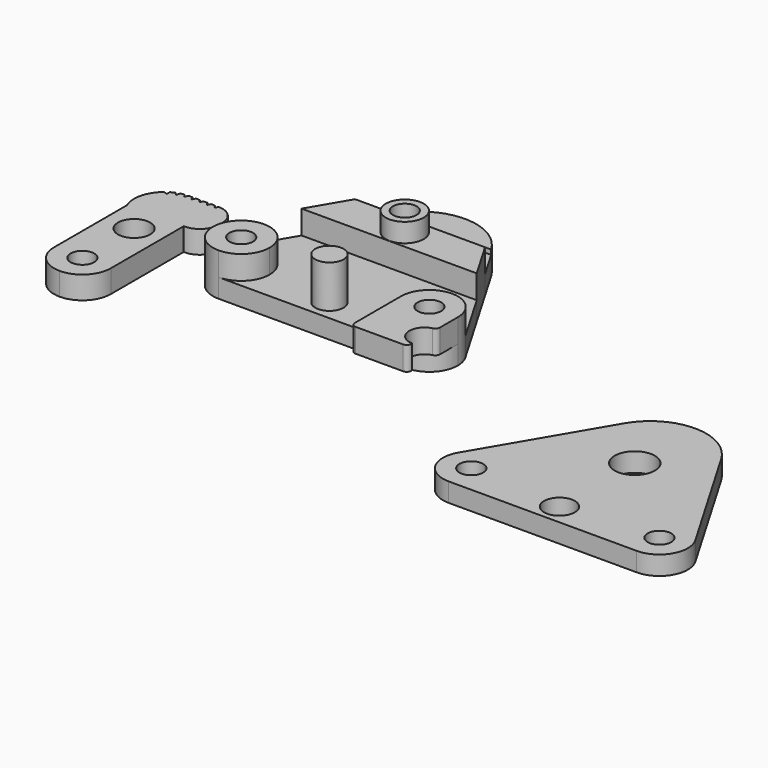
from build123d import *

# Parameters (mm, degrees)
F0_R            = 3.81
F2_DEPTH        = 5.08
F0_R_2          = 5.08
F0_R_3          = 3.175
F3_DEPTH        = 11.43
F4_DEPTH        = 16.51
F5_DEPTH        = 6.35
F6_START        = 5.08
F6_DEPTH        = 6.35
F1_R            = 3.175
F1_R_2          = 4.318
F7_DEPTH        = 6.096
F8_R            = 3.175
F8_R_2          = 4.1275
F8_R_3          = 5.3975
F9_DEPTH        = 5.08
F10_D           = 6.35
F10_CBORE_D     = 12.7
F10_CBORE_DEPTH = 3.81


# Not quite as in the source:
# - a feature names something its author has since deleted; it is built from what else it names


with BuildPart() as f2:
    # F0 (on Top) → F2 (new body)
    with BuildSketch(Plane.XY):
        with BuildLine():
            ThreePointArc((-17.6954780992, -30.626333441), (-19.9273244266, -36.0144871136), (-25.3154780992, -38.246333441))
            Line((-25.3154780992, -38.246333441), (17.5577984688, -38.246333441))
            Line((17.5577984688, -38.246333441), (17.5577984688, -30.626333441))
            ThreePointArc((17.5577984688, -30.626333441), (23.1855190024, -23.271387994), (31.7560196047, -26.7803736534))
            Line((31.7560196047, -26.7803736534), (23.4553135122, -12.5826484363))
            Line((23.4553135122, -12.5826484363), (-23.5570166859, -12.5826484363))
            Line((-23.5570166859, -12.5826484363), (-31.8864294526, -26.7679661294))
            ThreePointArc((-31.8864294526, -26.7679661294), (-23.3162594159, -23.2732711771), (-17.6954780992, -30.626333441))
        make_face()
        with Locations((0, -32.6841548085)):
            Circle(F0_R, mode=Mode.SUBTRACT)
        with BuildLine():
            Line((17.5577984688, -30.626333441), (17.5577984688, -38.246333441))
            Line((17.5577984688, -38.246333441), (25.1777984688, -38.246333441))
            ThreePointArc((25.1777984688, -38.246333441), (19.7896447962, -36.0144871136), (17.5577984688, -30.626333441))
        make_face()
    extrude(amount=F2_DEPTH)



with BuildPart() as f2b:
    # F0 (on Top) → F2, piece 2 (new body)
    with BuildSketch(Plane.XY):
        Polygon((-13.0052492681, 5.3874266745), (-17.4796027267, -2.2325733255), (17.4113143411, -2.2448484363), (12.9634277073, 5.3629227003), align=None)
    extrude(amount=F2_DEPTH)


with BuildPart() as f2_1:
    add(f2.part)

    add(f2b.part)  # F3 merges F2b
    # F0 (on Top) → F3 (join)
    with BuildSketch(Plane.XY):
        Polygon((-17.4796027267, -2.2325733255), (-23.5570166859, -12.5826484363), (23.4553135122, -12.5826484363), (17.4113143411, -2.2448484363), align=None)
        with Locations((0, -7.4137484363)):
            Circle(F0_R_2, mode=Mode.SUBTRACT)
        with BuildLine():
            ThreePointArc((-31.8864294526, -26.7679661294), (-31.9285393765, -34.4120725422), (-25.3154780992, -38.246333441))
            ThreePointArc((-25.3154780992, -38.246333441), (-19.9273244266, -36.0144871136), (-17.6954780992, -30.626333441))
            ThreePointArc((-17.6954780992, -30.626333441), (-23.3162594159, -23.2732711771), (-31.8864294526, -26.7679661294))
        make_face()
        with Locations((-25.3154780992, -30.626333441)):
            Circle(F0_R_3, mode=Mode.SUBTRACT)
        with BuildLine():
            ThreePointArc((17.5577984688, -30.626333441), (19.7896447962, -36.0144871136), (25.1777984688, -38.246333441))
            ThreePointArc((25.1777984688, -38.246333441), (30.5659521415, -36.0144871136), (32.7977984688, -30.626333441))
            ThreePointArc((32.7977984688, -30.626333441), (32.5327439158, -28.6340539746), (31.7560196047, -26.7803736534))
            ThreePointArc((31.7560196047, -26.7803736534), (23.1855190024, -23.271387994), (17.5577984688, -30.626333441))
        make_face()
        with Locations((25.1777984688, -30.626333441)):
            Circle(F0_R_3, mode=Mode.SUBTRACT)
        with BuildLine():
            Line((17.5577984688, -30.626333441), (17.5577984688, -38.246333441))
            Line((17.5577984688, -38.246333441), (25.1777984688, -38.246333441))
            ThreePointArc((25.1777984688, -38.246333441), (19.7896447962, -36.0144871136), (17.5577984688, -30.626333441))
        make_face()
        with Locations((25.1777984688, -30.626333441)):
            Circle(F0_R_3)
        with Locations((-25.3154780992, -30.626333441)):
            Circle(F0_R_3)
    extrude(amount=F3_DEPTH)

    # F0 (on Top) → F4 (join)
    with BuildSketch(Plane.XY):
        with Locations((0, -32.6841548085)):
            Circle(F0_R)
        with Locations((0, -7.4137484363)):
            Circle(F0_R_2)
        with Locations((0, -7.4137484363)):
            Circle(F0_R_3, mode=Mode.SUBTRACT)
        with Locations((0, -7.4137484363)):
            Circle(F0_R_3)
    extrude(amount=F4_DEPTH)

    # F0 (on Top) → F5 (join)
    with BuildSketch(Plane.XY):
        with BuildLine():
            ThreePointArc((12.9634277073, 5.3629227003), (-0.0138892827, 12.8163759997), (-13.0052492681, 5.3874266745))
            Line((-13.0052492681, 5.3874266745), (12.9634277073, 5.3629227003))
        make_face()
    extrude(amount=F5_DEPTH)

    # F0 (on Top) → F6 (join)
    with BuildSketch(Plane.XY.offset(F6_START)):
        with BuildLine():
            Line((25.1777984688, -38.246333441), (17.5577984688, -38.246333441))
            Line((17.5577984688, -38.246333441), (17.5577984688, -46.1423077567))
            ThreePointArc((17.5577984688, -46.1423077567), (17.9297728567, -47.0403333688), (18.8277984688, -47.4123077567))
            Line((18.8277984688, -47.4123077567), (31.5277984688, -47.4123077567))
            ThreePointArc((31.5277984688, -47.4123077567), (32.4258240809, -47.0403333688), (32.7977984688, -46.1423077567))
            Line((32.7977984688, -46.1423077567), (32.7977984688, -46.0876021411))
            ThreePointArc((32.7977984688, -46.0876021411), (32.7285996668, -45.9133479668), (32.5587077819, -45.8340400927))
            ThreePointArc((32.5587077819, -45.8340400927), (28.7412851246, -42.1364642502), (31.8296571838, -37.8113352487))
            ThreePointArc((31.8296571838, -37.8113352487), (32.5268631734, -37.3618027602), (32.7977984688, -36.5777302406))
            Line((32.7977984688, -36.5777302406), (32.7977984688, -30.626333441))
            ThreePointArc((32.7977984688, -30.626333441), (30.5659521415, -36.0144871136), (25.1777984688, -38.246333441))
        make_face()
    extrude(amount=F6_DEPTH)

    # F10 (through all)
    with Locations(Plane(origin=(0, 0, 0), x_dir=(1, 0, 0), z_dir=(0, 0, -1))):
        with Locations((-25.3154780992, 30.626333441), (25.1777984688, 30.626333441), (0, 7.4137484363)):
            CounterBoreHole(F10_D / 2, F10_CBORE_D / 2, F10_CBORE_DEPTH)


with BuildPart() as f7:
    # F1 (on face) → F7 (new body)
    with BuildSketch(Plane.XY):
        with BuildLine():
            ThreePointArc((-57.1931454593, -16.6974549338), (-59.9398799438, -21.0814893724), (-59.5037853794, -26.2364995391))
            Line((-59.5037853794, -26.2364995391), (-44.4651611469, -26.2364995391))
            Line((-44.4651611469, -26.2364995391), (-44.2637853794, -26.2364995391))
            Line((-44.2637853794, -26.2364995391), (-44.0075451514, -26.2364995391))
            ThreePointArc((-44.0075451514, -26.2364995391), (-40.415442703, -24.7486019875), (-38.9275451514, -21.1564995391))
            Line((-38.9275451514, -21.1564995391), (-38.9275451514, -19.9137048024))
            ThreePointArc((-38.9275451514, -19.9137048024), (-40.4075319267, -16.3295305904), (-43.9851454593, -14.8337541872))
            Line((-43.9851454593, -14.8337541872), (-44.4931882277, -15.7136113037))
            Line((-44.4931882277, -15.7136113037), (-45.0011454593, -14.8337048024))
            Line((-45.0011454593, -14.8337048024), (-46.0171454593, -14.8337048024))
            Line((-46.0171454593, -14.8337048024), (-46.5251454593, -15.7135866127))
            Line((-46.5251454593, -15.7135866127), (-47.0331454593, -14.8337048024))
            Line((-47.0331454593, -14.8337048024), (-48.0491454593, -14.8337048024))
            Line((-48.0491454593, -14.8337048024), (-48.5571454593, -15.7135866127))
            Line((-48.5571454593, -15.7135866127), (-49.0651454593, -14.8337048024))
            Line((-49.0651454593, -14.8337048024), (-50.0811454593, -14.8337048024))
            Line((-50.0811454593, -14.8337048024), (-50.5891454593, -15.7135866127))
            Line((-50.5891454593, -15.7135866127), (-51.0971454593, -14.8337048024))
            Line((-51.0971454593, -14.8337048024), (-51.7384644685, -14.8337048024))
            Line((-51.7384644685, -14.8337048024), (-52.1131454593, -14.8337048024))
            Line((-52.1131454593, -14.8337048024), (-52.5538799272, -15.7491331879))
            Line((-52.5538799272, -15.7491331879), (-53.1291454593, -14.9116813579))
            ThreePointArc((-53.1291454593, -14.9116813579), (-53.6404575982, -14.9998355114), (-54.1451454593, -15.120257357))
            Line((-54.1451454593, -15.120257357), (-54.3722812556, -16.1105428361))
            Line((-54.3722812556, -16.1105428361), (-55.1611454593, -15.4702700285))
            ThreePointArc((-55.1611454593, -15.4702700285), (-55.6780776214, -15.7088475189), (-56.1771454593, -15.9828354243))
            Line((-56.1771454593, -15.9828354243), (-56.2225596223, -16.9978199334))
            Line((-56.2225596223, -16.9978199334), (-57.1931454593, -16.6974549338))
        make_face()
        with BuildLine():
            Line((-44.4651611469, -26.2364995391), (-59.5037853794, -26.2364995391))
            Line((-59.5037853794, -26.2364995391), (-59.5037853794, -50.714222083))
            ThreePointArc((-59.5037853794, -50.714222083), (-57.271939052, -56.1023757557), (-51.8837853794, -58.334222083))
            ThreePointArc((-51.8837853794, -58.334222083), (-46.4956317067, -56.1023757557), (-44.2637853794, -50.714222083))
            Line((-44.2637853794, -50.714222083), (-44.2637853794, -26.2364995391))
            Line((-44.2637853794, -26.2364995391), (-44.4651611469, -26.2364995391))
        make_face()
        with Locations((-51.8837853794, -50.714222083)):
            Circle(F1_R, mode=Mode.SUBTRACT)
        with Locations((-51.7384644685, -33.5519946396)):
            Circle(F1_R_2, mode=Mode.SUBTRACT)
    extrude(amount=F7_DEPTH)


with BuildPart() as f9:
    # F8 (on Top) → F9 (new body)
    with BuildSketch(Plane.XY):
        with BuildLine():
            ThreePointArc((63.6413138902, -68.9986979613), (63.5992039663, -76.6428043742), (70.2122652436, -80.4770652729))
            Line((70.2122652436, -80.4770652729), (120.7055418116, -80.4770652729))
            ThreePointArc((120.7055418116, -80.4770652729), (127.3150279331, -76.649042753), (127.2837629474, -69.0111054854))
            Line((127.2837629474, -69.0111054854), (108.4911710501, -36.8678091316))
            ThreePointArc((108.4911710501, -36.8678091316), (95.5138540601, -29.4143558323), (82.5224940747, -36.8433051574))
            Line((82.5224940747, -36.8433051574), (63.6413138902, -68.9986979613))
        make_face()
        with Locations((70.2122652436, -72.8570652729)):
            Circle(F8_R, mode=Mode.SUBTRACT)
        with Locations((95.5277433428, -74.9148866405)):
            Circle(F8_R_2, mode=Mode.SUBTRACT)
        with Locations((120.7055418116, -72.8570652729)):
            Circle(F8_R, mode=Mode.SUBTRACT)
        with Locations((95.5277433428, -49.6444802682)):
            Circle(F8_R_3, mode=Mode.SUBTRACT)
    extrude(amount=F9_DEPTH)


solid = Compound([f2_1.part, f7.part, f9.part])
